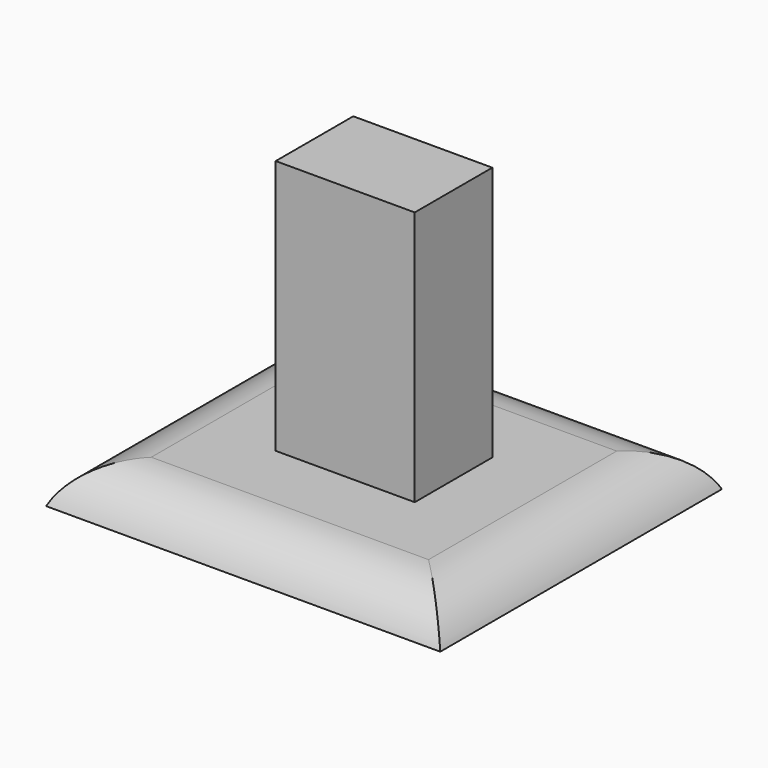
from build123d import *

# Parameters (mm, degrees)
F0_W        = 10.9
F0_H        = 7.6
F1_DEPTH    = 20
F2_W        = 30.9
F2_H        = 27.6
F2_W_2      = 10.9
F2_H_2      = 7.6
F3_DEPTH    = 3
F4_T1_DEPTH = 50.5128784748
F4_T3_DEPTH = 53.8128784748


# Not quite as in the source:
# - a fillet or chamfer that OpenCascade refuses, or shapes differently, is made with other operations: its cross-section is extruded or revolved along the edge and cut away or added


with BuildPart() as f1:
    # F0 (on Top) → F1 (new body)
    with BuildSketch(Plane.XY):
        with Locations((1.5206737995, 10.1067991287)):
            Rectangle(F0_W, F0_H)
    extrude(amount=F1_DEPTH)

    # F2 (on face) → F3 (join)
    with BuildSketch(Plane(origin=(0, 0, 0), x_dir=(1, 0, 0), z_dir=(0, 0, -1))):
        with Locations((1.5206737995, -10.1067991287)):
            Rectangle(F2_W, F2_H)
        with Locations((1.5206737995, -10.1067991287)):
            Rectangle(F2_W_2, F2_H_2, mode=Mode.SUBTRACT)
        with Locations((1.5206737995, -10.1067991287)):
            Rectangle(F2_W_2, F2_H_2)
    extrude(amount=F3_DEPTH)

    # F4: fillet of radius 5 on 4 edges, made by hand

    # F4_s2 → F4_t1 (cut)
    with BuildSketch(Plane.XZ.offset(-35.363238366)):
        with BuildLine():
            ThreePointArc((-13.9293262005, -3), (-12.0853632931, -0.8166998673), (-9.3467505055, 0))
            Line((-9.3467505055, 0), (-13.9293262005, 0))
            Line((-13.9293262005, 0), (-13.9293262005, -3))
        make_face()
        with BuildLine():
            ThreePointArc((12.3880981046, 0), (15.1267108921, -0.8166998673), (16.9706737995, -3))
            Line((16.9706737995, -3), (16.9706737995, 0))
            Line((16.9706737995, 0), (12.3880981046, 0))
        make_face()
    extrude(amount=F4_T1_DEPTH, mode=Mode.SUBTRACT)

    # F4_s4 → F4_t3 (cut)
    with BuildSketch(Plane.YZ.offset(-25.3857654379)):
        with BuildLine():
            ThreePointArc((-3.6932008713, -3), (-1.8492379639, -0.8166998673), (0.8893748236, 0))
            Line((0.8893748236, 0), (-3.6932008713, 0))
            Line((-3.6932008713, 0), (-3.6932008713, -3))
        make_face()
        with BuildLine():
            ThreePointArc((23.9067991287, -3), (22.0628362212, -0.8166998673), (19.3242234337, 0))
            Line((19.3242234337, 0), (23.9067991287, 0))
            Line((23.9067991287, 0), (23.9067991287, -3))
        make_face()
    extrude(amount=F4_T3_DEPTH, mode=Mode.SUBTRACT)


solid = f1.part
